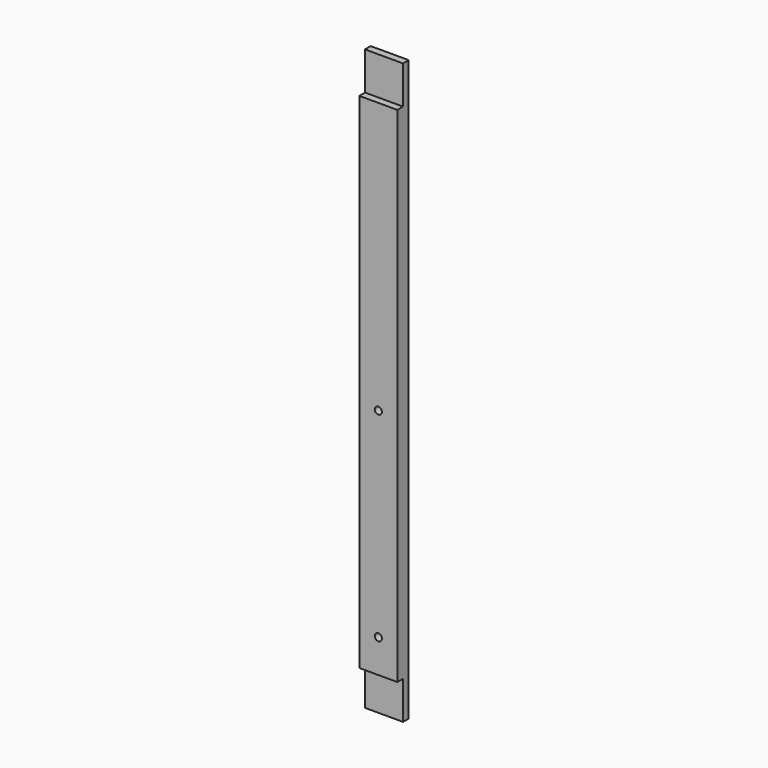
from build123d import *

# Parameters (mm, degrees)
F0_W     = 50.8
F0_H     = 19.05
F1_DEPTH = 774.7
F2_W     = 122.43557321
F2_H     = 50.8
F2_W_2   = 343.1604206562
F3_DEPTH = 25.4
F4_R     = 0.79375
F5_DEPTH = 25.4
F6_R     = 4.7625
F7_DEPTH = 25.4


# Not quite as in the source:
# - a feature names something its author has since deleted; it is built from what else it names


with BuildPart() as f1:
    # F0 (on Top) → F1 (new body)
    with BuildSketch(Plane.XY):
        Rectangle(F0_W, F0_H)
    extrude(amount=F1_DEPTH)

    # F2 (on Front) → F3 (cut)
    with BuildSketch(Plane.XZ):
        with Locations((22.4465244144, 25.4)):
            Rectangle(F2_W, F2_H)
        with Locations((-38.7818217278, 749.3)):
            Rectangle(F2_W_2, F2_H)
    extrude(amount=F3_DEPTH, mode=Mode.SUBTRACT)

    # F4 (on Front) → F5 (cut)
    with BuildSketch(Plane.XZ):
        with Locations((9.525, 101.6)):
            Circle(F4_R)
        with Locations((9.525, 155.575)):
            Circle(F4_R)
        with Locations((9.525, 619.125)):
            Circle(F4_R)
        with Locations((9.525, 673.1)):
            Circle(F4_R)
        with Locations((-9.525, 619.125)):
            Circle(F4_R)
        with Locations((-9.525, 673.1)):
            Circle(F4_R)
        with Locations((-9.525, 101.6)):
            Circle(F4_R)
        with Locations((-9.525, 155.575)):
            Circle(F4_R)
    extrude(amount=-F5_DEPTH, mode=Mode.SUBTRACT)

    # F6 (on Front) → F7 (cut)
    with BuildSketch(Plane.XZ):
        with Locations((0, 95.25)):
            Circle(F6_R)
        with Locations((0, 361.95)):
            Circle(F6_R)
    extrude(amount=F7_DEPTH, mode=Mode.SUBTRACT)


solid = f1.part
